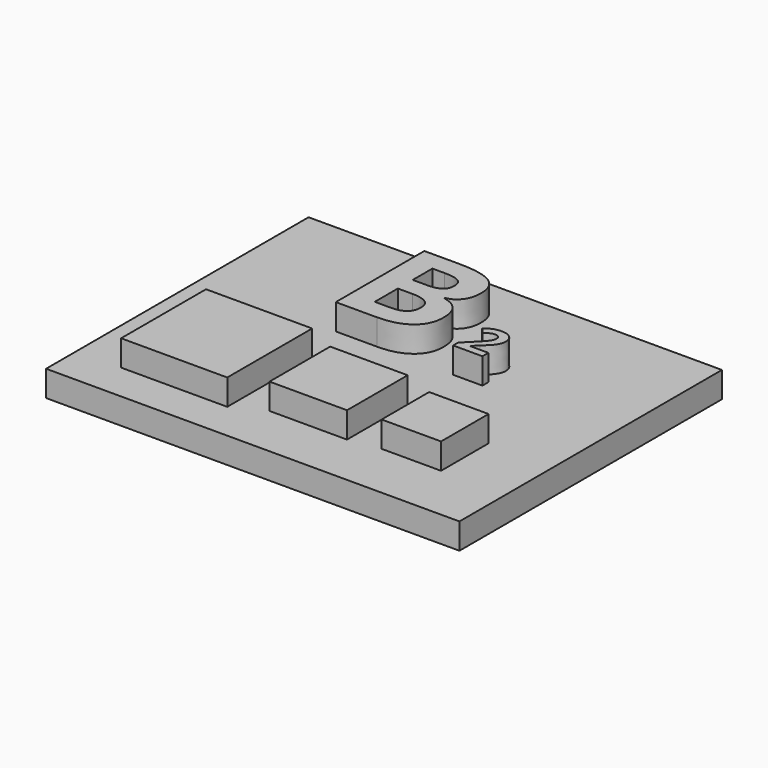
from build123d import *

# Parameters (mm, degrees)
F1_W           = 20.5434848444
F1_H           = 20.5434804712
F1_W_2         = 15
F1_H_2         = 14.6739158718
F1_W_3         = 11.5
F1_H_3         = 11.5
F1_TEXT_SIZE   = 11.3546977647
F1_TEXT_SIZE_2 = 30.0088431686
F2_DEPTH       = 10
F3_DEPTH       = 5


# Not quite as in the source:
# - a feature names something its author has since deleted; it is built from what else it names
# - Text() gives the source's letters only with a copy of the font that has no kerning and outlines rounded to 1/6400 em; it was checked with that copy


with BuildPart() as f2:
    # F1 (on Top) → F2 (new body)
    with BuildSketch(Plane.XY):
        with Locations((-21.1021756343, -15.8611078782)):
            Rectangle(F1_W, F1_H)
        with Locations((2.4999999441, -15.8611079156)):
            Rectangle(F1_W_2, F1_H_2)
        with Locations((21.7246557474, -16.5446088761)):
            Rectangle(F1_W_3, F1_H_3)
        with Locations((8.8221495971, 3.3776834607)):
            Text('2', F1_TEXT_SIZE, font='Open Sans', font_style=FontStyle.BOLD, text_align=(TextAlign.LEFT, TextAlign.BOTTOM))
        with Locations((-16.1319971085, 3.3776834607)):
            Text('B', F1_TEXT_SIZE_2, font='Open Sans', font_style=FontStyle.BOLD, text_align=(TextAlign.LEFT, TextAlign.BOTTOM))
    extrude(amount=F2_DEPTH)

    # F0 (on Top) → F3 (join)
    with BuildSketch(Plane.XY):
        Polygon((-40, -33.5), (40, -33.5), (40, -32.5), (40, -30), (40, 30), (-40, 30), (-40, -30), (-40, -32.5), align=None)
    extrude(amount=F3_DEPTH)


solid = f2.part
